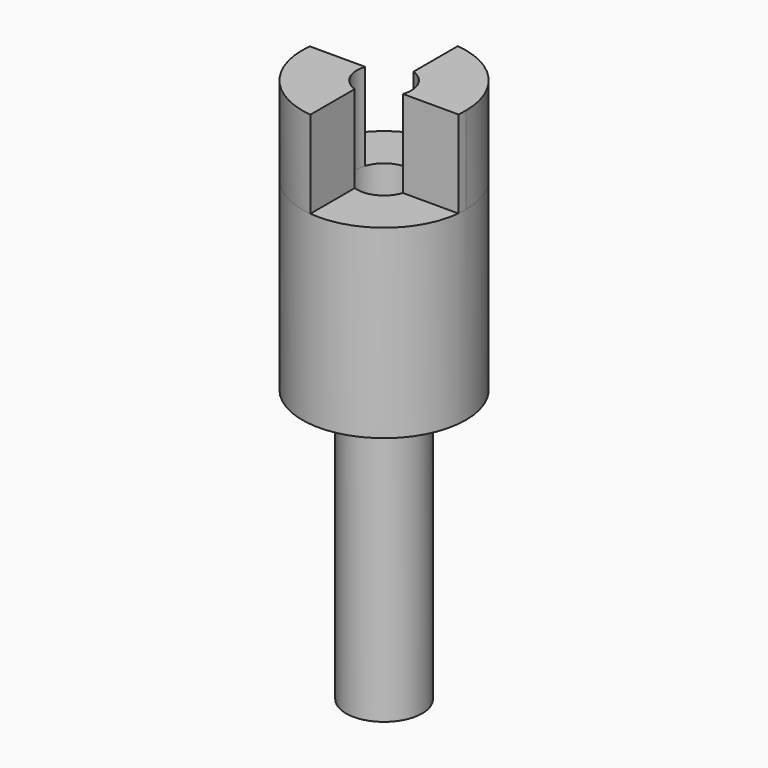
from build123d import *

# Parameters (mm, degrees)
F3_DEPTH = 8


# Not quite as in the source:
# - after a boolean that leaves OpenCascade's solid faulty, fix() repairs it


with BuildPart() as f1:
    # F0 (on Front) → F1 (revolve)
    with BuildSketch(Plane.XZ):
        Polygon((2.5, 5), (0, 5), (0, -25), (3.5, -25), (3.5, 0), (7.5, 0), (7.5, 17), (2.5, 17), align=None)
    revolve(axis=Axis((0, 0, -10), (0, 0, -1)))

    # F2 (on face) → F3 (join)
    with BuildSketch(Plane.XY.offset(17)):
        with BuildLine():
            ThreePointArc((7.5, 0), (5.5789784011, 5.0124844139), (0.8, 7.457211275))
            Line((0.8, 7.457211275), (0.8, 2.3685438565))
            ThreePointArc((0.8, 2.3685438565), (2.0310096012, 1.4577379737), (2.5, 0))
            ThreePointArc((2.5, 0), (2.466917068, -0.4053642552), (2.3685438565, -0.8))
            Line((2.3685438565, -0.8), (7.457211275, -0.8))
            ThreePointArc((7.457211275, -0.8), (7.4892951792, -0.4005717398), (7.5, 0))
        make_face()
        with BuildLine():
            Line((-2.3685438565, 0.8), (-7.457211275, 0.8))
            ThreePointArc((-7.457211275, 0.8), (-5.8387300862, -4.7073592363), (-0.8, -7.457211275))
            Line((-0.8, -7.457211275), (-0.8, -2.3685438565))
            ThreePointArc((-0.8, -2.3685438565), (-2.2404988474, -1.1091279975), (-2.3685438565, 0.8))
        make_face()
    extrude(amount=F3_DEPTH)

    add(f1.part.fix(), mode=Mode.REPLACE)


solid = f1.part
